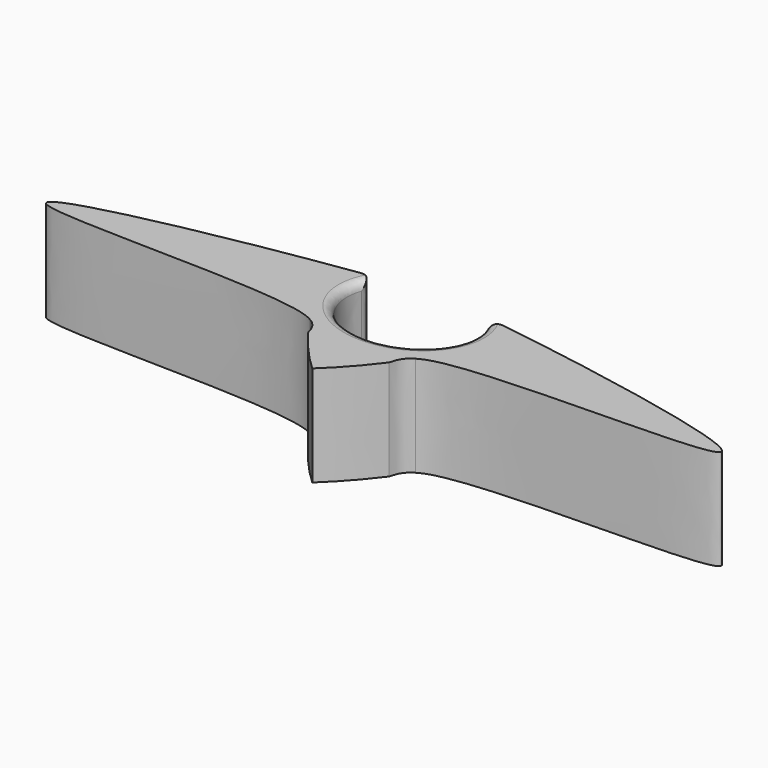
from build123d import *

# Parameters (mm, degrees)
F1_DEPTH = 19.05
F2_R     = 1.5875


with BuildPart() as f1:
    # F0 (on Top) → F1 (new body)
    with BuildSketch(Plane.XY):
        with BuildLine():
            add(Edge.make_bspline(
                [(12.192, 0), (12.7223990452, -1.6113208548), (13.4528032472, -4.9234335968), (10.9542579474, -9.8536995693), (9.9912040784, -11.4268014978)],
                knots=[0, 0, 0, 0, 0.3681337258, 0.5332552828, 0.5332552828, 0.5332552828, 0.5332552828], degree=3))
            add(Edge.make_bspline(
                [(-12.192, 0), (-12.192, -10.3124), (0, -10.3124), (12.192, -10.3124), (12.192, 0)],
                knots=[3.1415926536, 3.1415926536, 3.1415926536, 4.7123889804, 4.7123889804, 6.2831853072, 6.2831853072, 6.2831853072], degree=2, weights=[1, 0.7071067812, 1, 0.7071067812, 1]))
            add(Edge.make_bspline(
                [(-12.192, 0), (-12.7223990452, -1.6113208548), (-13.4528032472, -4.9234335968), (-10.9542579474, -9.8536995693), (-9.9912040784, -11.4268014978)],
                knots=[0, 0, 0, 0, 0.3681337258, 0.5332552828, 0.5332552828, 0.5332552828, 0.5332552828], degree=3))
            add(Edge.make_bspline(
                [(-7.6780028803, -14.8338868503), (-8.0087573086, -13.6412017927), (-8.3425342331, -12.4180738358), (-9.9912040784, -11.4268014978)],
                knots=[0, 0, 0, 0, 0.1092981662, 0.1092981662, 0.1092981662, 0.1092981662], degree=3))
            add(Edge.make_bspline(
                [(-7.6780028803, -14.8338868503), (-5.2024397233, -18.1782384489), (-2.2659232737, -21.3830786791), (0, -23.4252623907)],
                knots=[0.651361281, 0.651361281, 0.651361281, 0.651361281, 1, 1, 1, 1], degree=3))
            add(Edge.make_bspline(
                [(7.6780028803, -14.8338868503), (5.2024397233, -18.1782384489), (2.2659232737, -21.3830786791), (0, -23.4252623907)],
                knots=[0.651361281, 0.651361281, 0.651361281, 0.651361281, 1, 1, 1, 1], degree=3))
            add(Edge.make_bspline(
                [(7.6780028803, -14.8338868503), (8.0087573086, -13.6412017927), (8.3425342331, -12.4180738358), (9.9912040784, -11.4268014978)],
                knots=[0, 0, 0, 0, 0.1092981662, 0.1092981662, 0.1092981662, 0.1092981662], degree=3))
        make_face()
        with BuildLine():
            add(Edge.make_bspline(
                [(12.192, 0), (12.192, 2.9234439961), (10.3781378892, 5.4119532564)],
                knots=[0, 0, 0, 0.5524807942, 0.5524807942, 0.5524807942], degree=2, weights=[1, 0.9620876313, 1]))
            add(Edge.make_bspline(
                [(12.192, 0), (12.7223990452, -1.6113208548), (13.4528032472, -4.9234335968), (10.9542579474, -9.8536995693), (9.9912040784, -11.4268014978)],
                knots=[0, 0, 0, 0, 0.3681337258, 0.5332552828, 0.5332552828, 0.5332552828, 0.5332552828], degree=3))
            add(Edge.make_bspline(
                [(9.9912040784, -11.4268014978), (10.5541126942, -11.088349417), (19.3390054034, -7.2684023777), (96.5968069209, -10.8050176336), (38.7669496827, 1.4617408009), (10.3781378892, 5.4119532564)],
                knots=[0.1092981662, 0.1092981662, 0.1092981662, 0.1092981662, 0.1466160559, 0.5670428182, 1, 1, 1, 1], degree=3))
        make_face()
        with BuildLine():
            add(Edge.make_bspline(
                [(-12.192, 0), (-12.7223990452, -1.6113208548), (-13.4528032472, -4.9234335968), (-10.9542579474, -9.8536995693), (-9.9912040784, -11.4268014978)],
                knots=[0, 0, 0, 0, 0.3681337258, 0.5332552828, 0.5332552828, 0.5332552828, 0.5332552828], degree=3))
            add(Edge.make_bspline(
                [(-10.3781378892, 5.4119532564), (-12.192, 2.9234439961), (-12.192, 0)],
                knots=[2.5891118594, 2.5891118594, 2.5891118594, 3.1415926536, 3.1415926536, 3.1415926536], degree=2, weights=[1, 0.9620876313, 1]))
            add(Edge.make_bspline(
                [(-9.9912040784, -11.4268014978), (-10.5541126942, -11.088349417), (-19.3390054034, -7.2684023777), (-96.5968069209, -10.8050176336), (-38.7669496827, 1.4617408009), (-10.3781378892, 5.4119532564)],
                knots=[0.1092981662, 0.1092981662, 0.1092981662, 0.1092981662, 0.1466160559, 0.5670428182, 1, 1, 1, 1], degree=3))
        make_face()
    extrude(amount=F1_DEPTH)

    # F2
    f2_edges = [f1.edges().sort_by_distance(p)[0] for p in [
        (0, -10.3124, 19.05),
        (-10.378138, 5.411953, 9.525),
        (10.378138, 5.411953, 9.525),
        (0, -10.3124, 0),
    ]]
    fillet(f2_edges, radius=F2_R)


solid = f1.part
